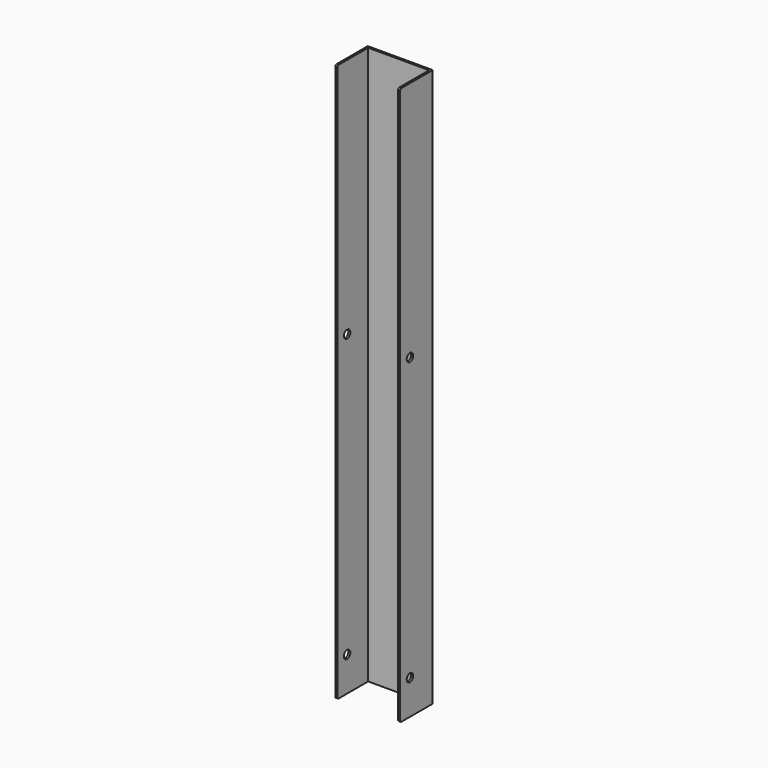
from build123d import *

# Parameters (mm, degrees)
F0_W     = 60
F0_H     = 550
F1_DEPTH = 2
F2_W     = 38
F2_H     = 550
F2_W_2   = 2
F3_DEPTH = 2
F4_W     = 38
F4_H     = 550
F4_W_2   = 2
F5_DEPTH = 2
F6_R     = 1.5
F7_R     = 1.5
F8_R     = 4
F9_DEPTH = 64.001


with BuildPart() as f1:
    # F0 (on Front) → F1 (new body)
    with BuildSketch(Plane.XZ):
        with Locations((-30, 275)):
            Rectangle(F0_W, F0_H)
    extrude(amount=-F1_DEPTH)

    # F2 (on face) → F3 (join)
    with BuildSketch(Plane.YZ):
        with Locations((-19, 275)):
            Rectangle(F2_W, F2_H)
        with Locations((1, 275)):
            Rectangle(F2_W_2, F2_H)
    extrude(amount=F3_DEPTH)

    # F4 (on face) → F5 (join)
    with BuildSketch(Plane(origin=(-60, 0, 0), x_dir=(0, -1, 0), z_dir=(-1, 0, 0))):
        with Locations((19, 275)):
            Rectangle(F4_W, F4_H)
        with Locations((-1, 275)):
            Rectangle(F4_W_2, F4_H)
    extrude(amount=F5_DEPTH)

    # F6
    f6_edges = [f1.edges().sort_by_distance(p)[0] for p in [
        (-61, -38, 0),
        (1, -38, 0),
    ]]
    fillet(f6_edges, radius=F6_R)

    # F7
    f7_edges = [f1.edges().sort_by_distance(p)[0] for p in [
        (-61, -38, 550),
        (1, -38, 550),
    ]]
    fillet(f7_edges, radius=F7_R)

    # F8 (on face) → F9 (cut, through all)
    with BuildSketch(Plane(origin=(-62, 0, 0), x_dir=(0, -1, 0), z_dir=(-1, 0, 0))):
        with Locations((26, 312)):
            Circle(F8_R)
        with Locations((26, 34)):
            Circle(F8_R)
    extrude(amount=-F9_DEPTH, mode=Mode.SUBTRACT)


solid = f1.part
